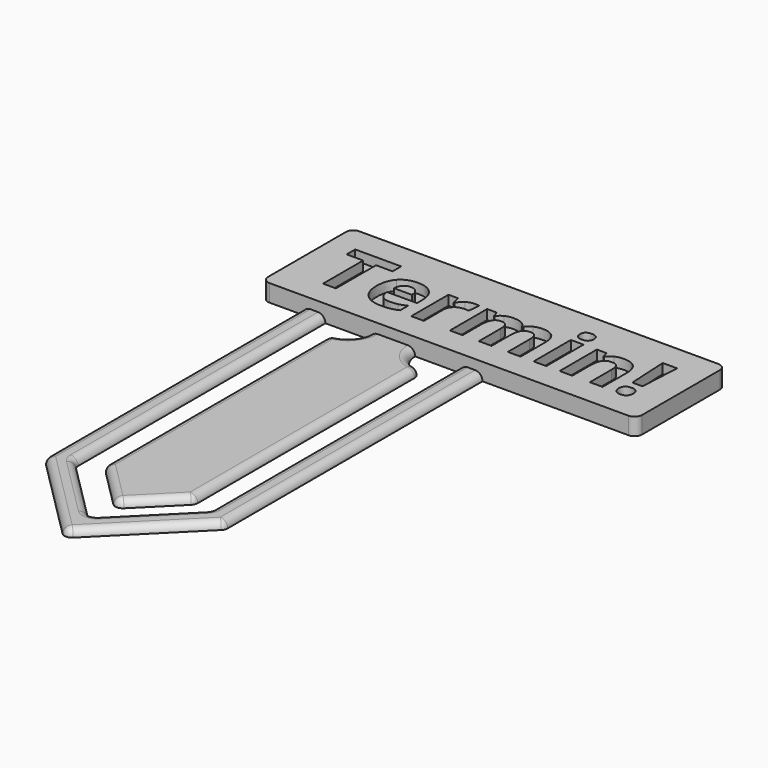
from build123d import *

# Parameters (mm, degrees)
F0_TEXT_SIZE = 11.3961958721
F1_DEPTH     = 1
F0_W         = 1.6969647916
F0_H         = 6.2216106839
F2_DEPTH     = 2.3
F3_R         = 0.99999


# Not quite as in the source:
# - a fillet or chamfer is up to 0.001 mm smaller than in the source, because OpenCascade refuses the exact size
# - Text() gives the source's letters only with a copy of the font that has no kerning and outlines rounded to 1/6400 em; it was checked with that copy


with BuildPart() as f1:
    # F0 (on Top) → F1 (new body)
    with BuildSketch(Plane.XY):
        Polygon((-11.1783012444, 18.0121831276), (-14.1783012444, 18.0121831276), (-14.1783012444, -24.9878168724), (-2.1783012444, -36.9878168724), (9.8216987556, -24.9878168724), (9.8216987556, 18.0121831276), (6.8216987556, 18.0121831276), (6.8216987556, -23.7451761852), (-2.1783012444, -32.7451761852), (-11.1783012444, -23.7451761852), align=None)
        with BuildLine():
            Line((0.8216987556, 18.0121831276), (-5.1783012444, 18.0121831276))
            ThreePointArc((-5.1783012444, 18.0121831276), (-6.0569809009, 15.8908627841), (-8.1783012444, 15.0121831276))
            Line((-8.1783012444, 15.0121831276), (-8.1783012444, -22.5025354981))
            Line((-8.1783012444, -22.5025354981), (-2.1783012444, -28.5025354981))
            Line((-2.1783012444, -28.5025354981), (3.8216987556, -22.5025354981))
            Line((3.8216987556, -22.5025354981), (3.8216987556, 15.0121831276))
            ThreePointArc((3.8216987556, 15.0121831276), (1.700378412, 15.8908627841), (0.8216987556, 18.0121831276))
        make_face()
        with Locations((-16.6529401391, 21.4095526137)):
            Text('Termin!', F0_TEXT_SIZE, font='Open Sans', font_style=FontStyle.BOLD, text_align=(TextAlign.LEFT, TextAlign.BOTTOM))
    extrude(amount=F1_DEPTH)

    # F0 (on Top) → F2 (join)
    with BuildSketch(Plane.XY):
        Polygon((-19.6529401391, 18.0121831276), (-14.1783012444, 18.0121831276), (-11.1783012444, 18.0121831276), (-5.1783012444, 18.0121831276), (0.8216987556, 18.0121831276), (6.8216987556, 18.0121831276), (9.8216987556, 18.0121831276), (30.3470598609, 18.0121831276), (30.3470598609, 33.0121831276), (-19.6529401391, 33.0121831276), align=None)
        Polygon((-12.4897673346, 28.1101596554), (-12.4897673346, 21.4095526137), (-14.2152226158, 21.4095526137), (-14.2152226158, 28.1101596554), (-16.4250162217, 28.1101596554), (-16.4250162217, 29.545368073), (-10.2817543843, 29.545368073), (-10.2817543843, 28.1101596554), align=None, mode=Mode.SUBTRACT)
        with BuildLine():
            add(Edge.make_bspline(
                [(-5.112511163, 21.4059913025), (-5.6182173548, 21.2973713106), (-6.3482861529, 21.2973713106)],
                knots=[0, 0, 0, 1, 1, 1], degree=2))
            add(Edge.make_bspline(
                [(-6.3482861529, 21.2973713106), (-7.8493788279, 21.2973713106), (-8.6951902403, 22.1271568225)],
                knots=[0, 0, 0, 1, 1, 1], degree=2))
            add(Edge.make_bspline(
                [(-8.6951902403, 22.1271568225), (-9.5410016527, 22.9569423344), (-9.5410016527, 24.4758415655)],
                knots=[0, 0, 0, 1, 1, 1], degree=2))
            add(Edge.make_bspline(
                [(-9.5410016527, 24.4758415655), (-9.5410016527, 26.0392571867), (-8.7592938421, 26.8930815493)],
                knots=[0, 0, 0, 1, 1, 1], degree=2))
            add(Edge.make_bspline(
                [(-8.7592938421, 26.8930815493), (-7.9775860314, 27.7469059119), (-6.5975779376, 27.7469059119)],
                knots=[0, 0, 0, 1, 1, 1], degree=2))
            add(Edge.make_bspline(
                [(-6.5975779376, 27.7469059119), (-5.2798927898, 27.7469059119), (-4.5453723528, 26.9963595744)],
                knots=[0, 0, 0, 1, 1, 1], degree=2))
            add(Edge.make_bspline(
                [(-4.5453723528, 26.9963595744), (-3.8108519157, 26.2458132369), (-3.8108519157, 24.9210054668)],
                knots=[0, 0, 0, 1, 1, 1], degree=2))
            Line((-3.8108519157, 24.9210054668), (-3.8108519157, 24.0965619217))
            Line((-3.8108519157, 24.0965619217), (-7.8226689938, 24.0965619217))
            add(Edge.make_bspline(
                [(-7.8226689938, 24.0965619217), (-7.7941785041, 23.373615746), (-7.393530993, 22.9676262681)],
                knots=[0, 0, 0, 1, 1, 1], degree=2))
            add(Edge.make_bspline(
                [(-7.393530993, 22.9676262681), (-6.9928834819, 22.5616367901), (-6.2699373062, 22.5616367901)],
                knots=[0, 0, 0, 1, 1, 1], degree=2))
            add(Edge.make_bspline(
                [(-6.2699373062, 22.5616367901), (-5.7072501351, 22.5616367901), (-5.20688591, 22.6782697323)],
                knots=[0, 0, 0, 1, 1, 1], degree=2))
            add(Edge.make_bspline(
                [(-5.20688591, 22.6782697323), (-4.706521685, 22.7949026744), (-4.1616410699, 23.0513170815)],
                knots=[0, 0, 0, 1, 1, 1], degree=2))
            Line((-4.1616410699, 23.0513170815), (-4.1616410699, 21.737193245))
            add(Edge.make_bspline(
                [(-4.1616410699, 21.737193245), (-4.6068049711, 21.5146112944), (-5.112511163, 21.4059913025)],
                knots=[0, 0, 0, 1, 1, 1], degree=2))
        make_face(mode=Mode.SUBTRACT)
        with BuildLine():
            add(Edge.make_bspline(
                [(-0.0296297384, 27.4272782308), (0.4627215363, 27.7469059119), (1.041434608, 27.7469059119)],
                knots=[0, 0, 0, 1, 1, 1], degree=2))
            add(Edge.make_bspline(
                [(1.041434608, 27.7469059119), (1.3868817953, 27.7469059119), (1.6148057128, 27.697047555)],
                knots=[0, 0, 0, 1, 1, 1], degree=2))
            Line((1.6148057128, 27.697047555), (1.4865985092, 26.1069220997))
            add(Edge.make_bspline(
                [(1.4865985092, 26.1069220997), (1.280042459, 26.1621224235), (0.9862342842, 26.1621224235)],
                knots=[0, 0, 0, 1, 1, 1], degree=2))
            add(Edge.make_bspline(
                [(0.9862342842, 26.1621224235), (0.1742553283, 26.1621224235), (-0.279811851, 25.7445586841)],
                knots=[0, 0, 0, 1, 1, 1], degree=2))
            add(Edge.make_bspline(
                [(-0.279811851, 25.7445586841), (-0.7338790302, 25.3269949447), (-0.7338790302, 24.5755582794)],
                knots=[0, 0, 0, 1, 1, 1], degree=2))
            Line((-0.7338790302, 24.5755582794), (-0.7338790302, 21.4095526137))
            Line((-0.7338790302, 21.4095526137), (-2.4308438218, 21.4095526137))
            Line((-2.4308438218, 21.4095526137), (-2.4308438218, 27.6311632976))
            Line((-2.4308438218, 27.6311632976), (-1.145210475, 27.6311632976))
            Line((-1.145210475, 27.6311632976), (-0.8941380347, 26.5841378019))
            Line((-0.8941380347, 26.5841378019), (-0.8122278769, 26.5841378019))
            add(Edge.make_bspline(
                [(-0.8122278769, 26.5841378019), (-0.5219810132, 27.1076505497), (-0.0296297384, 27.4272782308)],
                knots=[0, 0, 0, 1, 1, 1], degree=2))
        make_face(mode=Mode.SUBTRACT)
        with BuildLine():
            Line((8.3136320989, 24.5310418893), (8.3136320989, 21.4095526137))
            Line((8.3136320989, 21.4095526137), (6.6166673073, 21.4095526137))
            Line((6.6166673073, 21.4095526137), (6.6166673073, 25.0438707035))
            add(Edge.make_bspline(
                [(6.6166673073, 25.0438707035), (6.6166673073, 25.7169585222), (6.3914143732, 26.0535024316)],
                knots=[0, 0, 0, 1, 1, 1], degree=2))
            add(Edge.make_bspline(
                [(6.3914143732, 26.0535024316), (6.1661614392, 26.3900463409), (5.6818231146, 26.3900463409)],
                knots=[0, 0, 0, 1, 1, 1], degree=2))
            add(Edge.make_bspline(
                [(5.6818231146, 26.3900463409), (5.0301031632, 26.3900463409), (4.7354046606, 25.9110499832)],
                knots=[0, 0, 0, 1, 1, 1], degree=2))
            add(Edge.make_bspline(
                [(4.7354046606, 25.9110499832), (4.4407061579, 25.4320536254), (4.4407061579, 24.3369504283)],
                knots=[0, 0, 0, 1, 1, 1], degree=2))
            Line((4.4407061579, 24.3369504283), (4.4407061579, 21.4095526137))
            Line((4.4407061579, 21.4095526137), (2.7437413664, 21.4095526137))
            Line((2.7437413664, 21.4095526137), (2.7437413664, 27.6311632976))
            Line((2.7437413664, 27.6311632976), (4.0400586468, 27.6311632976))
            Line((4.0400586468, 27.6311632976), (4.2679825643, 26.8352102422))
            Line((4.2679825643, 26.8352102422), (4.3623573113, 26.8352102422))
            add(Edge.make_bspline(
                [(4.3623573113, 26.8352102422), (4.6134297516, 27.264348243), (5.0861938148, 27.5056270775)],
                knots=[0, 0, 0, 1, 1, 1], degree=2))
            add(Edge.make_bspline(
                [(5.0861938148, 27.5056270775), (5.5589578779, 27.7469059119), (6.171503406, 27.7469059119)],
                knots=[0, 0, 0, 1, 1, 1], degree=2))
            add(Edge.make_bspline(
                [(6.171503406, 27.7469059119), (7.5675374004, 27.7469059119), (8.0643403142, 26.8352102422)],
                knots=[0, 0, 0, 1, 1, 1], degree=2))
            Line((8.0643403142, 26.8352102422), (8.213915385, 26.8352102422))
            add(Edge.make_bspline(
                [(8.213915385, 26.8352102422), (8.4649878253, 27.2696902098), (8.9511068055, 27.5082980609)],
                knots=[0, 0, 0, 1, 1, 1], degree=2))
            add(Edge.make_bspline(
                [(8.9511068055, 27.5082980609), (9.4372257856, 27.7469059119), (10.0497713138, 27.7469059119)],
                knots=[0, 0, 0, 1, 1, 1], degree=2))
            add(Edge.make_bspline(
                [(10.0497713138, 27.7469059119), (11.1074807431, 27.7469059119), (11.6496903749, 27.2046962802)],
                knots=[0, 0, 0, 1, 1, 1], degree=2))
            add(Edge.make_bspline(
                [(11.6496903749, 27.2046962802), (12.1919000066, 26.6624866485), (12.1919000066, 25.4658860819)],
                knots=[0, 0, 0, 1, 1, 1], degree=2))
            Line((12.1919000066, 25.4658860819), (12.1919000066, 21.4095526137))
            Line((12.1919000066, 21.4095526137), (10.4895932482, 21.4095526137))
            Line((10.4895932482, 21.4095526137), (10.4895932482, 25.0438707035))
            add(Edge.make_bspline(
                [(10.4895932482, 25.0438707035), (10.4895932482, 25.7169585222), (10.2643403142, 26.0535024316)],
                knots=[0, 0, 0, 1, 1, 1], degree=2))
            add(Edge.make_bspline(
                [(10.2643403142, 26.0535024316), (10.0390873801, 26.3900463409), (9.5547490556, 26.3900463409)],
                knots=[0, 0, 0, 1, 1, 1], degree=2))
            add(Edge.make_bspline(
                [(9.5547490556, 26.3900463409), (8.9315195938, 26.3900463409), (8.6225758463, 25.9448824397)],
                knots=[0, 0, 0, 1, 1, 1], degree=2))
            add(Edge.make_bspline(
                [(8.6225758463, 25.9448824397), (8.3136320989, 25.4997185384), (8.3136320989, 24.5310418893)],
                knots=[0, 0, 0, 1, 1, 1], degree=2))
        make_face(mode=Mode.SUBTRACT)
        with Locations((14.7818635841, 24.5203579557)):
            Rectangle(F0_W, F0_H, mode=Mode.SUBTRACT)
        with BuildLine():
            add(Edge.make_bspline(
                [(14.7845345675, 28.4039678302), (13.8603743085, 28.4039678302), (13.8603743085, 29.239095309)],
                knots=[0, 0, 0, 1, 1, 1], degree=2))
            add(Edge.make_bspline(
                [(13.8603743085, 29.239095309), (13.8603743085, 30.0688808209), (14.7845345675, 30.0688808209)],
                knots=[0, 0, 0, 1, 1, 1], degree=2))
            add(Edge.make_bspline(
                [(14.7845345675, 30.0688808209), (15.7086948265, 30.0688808209), (15.7086948265, 29.239095309)],
                knots=[0, 0, 0, 1, 1, 1], degree=2))
            add(Edge.make_bspline(
                [(15.7086948265, 29.239095309), (15.7086948265, 28.8437897646), (15.4780999257, 28.6238787974)],
                knots=[0, 0, 0, 1, 1, 1], degree=2))
            add(Edge.make_bspline(
                [(15.4780999257, 28.6238787974), (15.2475050248, 28.4039678302), (14.7845345675, 28.4039678302)],
                knots=[0, 0, 0, 1, 1, 1], degree=2))
        make_face(mode=Mode.SUBTRACT)
        with BuildLine():
            add(Edge.make_bspline(
                [(24.9173552879, 21.507488672), (24.6618312085, 21.7549998011), (24.6618312085, 22.2055056691)],
                knots=[0, 0, 0, 1, 1, 1], degree=2))
            add(Edge.make_bspline(
                [(24.6618312085, 22.2055056691), (24.6618312085, 22.6720374376), (24.912013321, 22.9115356165)],
                knots=[0, 0, 0, 1, 1, 1], degree=2))
            add(Edge.make_bspline(
                [(24.912013321, 22.9115356165), (25.1621954335, 23.1510337954), (25.6411917913, 23.1510337954)],
                knots=[0, 0, 0, 1, 1, 1], degree=2))
            add(Edge.make_bspline(
                [(25.6411917913, 23.1510337954), (26.102381593, 23.1510337954), (26.3552346889, 22.9061936497)],
                knots=[0, 0, 0, 1, 1, 1], degree=2))
            add(Edge.make_bspline(
                [(26.3552346889, 22.9061936497), (26.6080877848, 22.661353504), (26.6080877848, 22.2055056691)],
                knots=[0, 0, 0, 1, 1, 1], degree=2))
            add(Edge.make_bspline(
                [(26.6080877848, 22.2055056691), (26.6080877848, 21.7656837347), (26.3525637055, 21.5128306388)],
                knots=[0, 0, 0, 1, 1, 1], degree=2))
            add(Edge.make_bspline(
                [(26.3525637055, 21.5128306388), (26.0970396262, 21.2599775429), (25.6411917913, 21.2599775429)],
                knots=[0, 0, 0, 1, 1, 1], degree=2))
            add(Edge.make_bspline(
                [(25.6411917913, 21.2599775429), (25.1728793672, 21.2599775429), (24.9173552879, 21.507488672)],
                knots=[0, 0, 0, 1, 1, 1], degree=2))
        make_face(mode=Mode.SUBTRACT)
        with BuildLine():
            Line((23.1536159111, 25.4658860819), (23.1536159111, 21.4095526137))
            Line((23.1536159111, 21.4095526137), (21.4566511195, 21.4095526137))
            Line((21.4566511195, 21.4095526137), (21.4566511195, 25.0438707035))
            add(Edge.make_bspline(
                [(21.4566511195, 25.0438707035), (21.4566511195, 25.7169585222), (21.2171529406, 26.0535024316)],
                knots=[0, 0, 0, 1, 1, 1], degree=2))
            add(Edge.make_bspline(
                [(21.2171529406, 26.0535024316), (20.9776547618, 26.3900463409), (20.4541420139, 26.3900463409)],
                knots=[0, 0, 0, 1, 1, 1], degree=2))
            add(Edge.make_bspline(
                [(20.4541420139, 26.3900463409), (19.7418797719, 26.3900463409), (19.4249230742, 25.9146112944)],
                knots=[0, 0, 0, 1, 1, 1], degree=2))
            add(Edge.make_bspline(
                [(19.4249230742, 25.9146112944), (19.1079663765, 25.4391762478), (19.1079663765, 24.3369504283)],
                knots=[0, 0, 0, 1, 1, 1], degree=2))
            Line((19.1079663765, 24.3369504283), (19.1079663765, 21.4095526137))
            Line((19.1079663765, 21.4095526137), (17.4110015849, 21.4095526137))
            Line((17.4110015849, 21.4095526137), (17.4110015849, 27.6311632976))
            Line((17.4110015849, 27.6311632976), (18.7073188654, 27.6311632976))
            Line((18.7073188654, 27.6311632976), (18.9352427828, 26.8352102422))
            Line((18.9352427828, 26.8352102422), (19.0296175299, 26.8352102422))
            add(Edge.make_bspline(
                [(19.0296175299, 26.8352102422), (19.3145224267, 27.2857161102), (19.8122156683, 27.5163110111)],
                knots=[0, 0, 0, 1, 1, 1], degree=2))
            add(Edge.make_bspline(
                [(19.8122156683, 27.5163110111), (20.3099089099, 27.7469059119), (20.9438223053, 27.7469059119)],
                knots=[0, 0, 0, 1, 1, 1], degree=2))
            add(Edge.make_bspline(
                [(20.9438223053, 27.7469059119), (22.0300222243, 27.7469059119), (22.5918190677, 27.1601798901)],
                knots=[0, 0, 0, 1, 1, 1], degree=2))
            add(Edge.make_bspline(
                [(22.5918190677, 27.1601798901), (23.1536159111, 26.5734538682), (23.1536159111, 25.4658860819)],
                knots=[0, 0, 0, 1, 1, 1], degree=2))
        make_face(mode=Mode.SUBTRACT)
        Polygon((26.6080877848, 29.545368073), (26.3249635436, 24.1090265109), (24.9681039726, 24.1090265109), (24.6831990758, 29.545368073), align=None, mode=Mode.SUBTRACT)
        with BuildLine():
            add(Edge.make_bspline(
                [(-5.7303986579, 26.1977355356), (-6.0473553556, 26.5396214117), (-6.5868940039, 26.5396214117)],
                knots=[0, 0, 0, 1, 1, 1], degree=2))
            add(Edge.make_bspline(
                [(-6.5868940039, 26.5396214117), (-7.1264326522, 26.5396214117), (-7.4327054163, 26.1977355356)],
                knots=[0, 0, 0, 1, 1, 1], degree=2))
            add(Edge.make_bspline(
                [(-7.4327054163, 26.1977355356), (-7.7389781804, 25.8558496594), (-7.7834945705, 25.2272782308)],
                knots=[0, 0, 0, 1, 1, 1], degree=2))
            Line((-7.7834945705, 25.2272782308), (-5.400977371, 25.2272782308))
            add(Edge.make_bspline(
                [(-5.400977371, 25.2272782308), (-5.4134419602, 25.8558496594), (-5.7303986579, 26.1977355356)],
                knots=[0, 0, 0, 1, 1, 1], degree=2))
        make_face()
    extrude(amount=F2_DEPTH)

    # F3 (radius 1 in the source; OpenCascade refuses exactly that, so slightly less here)
    f3_edges = [f1.edges().sort_by_distance(p)[0] for p in [
        (-19.65294, 18.012183, 1.15),
        (-19.65294, 33.012183, 1.15),
        (30.34706, 33.012183, 1.15),
        (30.34706, 18.012183, 1.15),
        (-2.178301, -36.987817, 0.5),
        (9.821699, -24.987817, 0.5),
        (-14.178301, -24.987817, 0.5),
        (-8.178301, -22.502535, 0.5),
        (-2.178301, -28.502535, 0.5),
        (3.821699, -22.502535, 0.5),
        (-8.178301, 15.012183, 0.5),
        (3.821699, 15.012183, 0.5),
        (3.821699, -30.987817, 1),
        (9.821699, -3.487817, 1),
        (-8.178301, -30.987817, 1),
        (-14.178301, -3.487817, 1),
        (3.821699, -3.745176, 1),
        (1.700378, 15.890863, 1),
        (-6.056981, 15.890863, 1),
        (-8.178301, -3.745176, 1),
        (-5.178301, -25.502535, 1),
        (0.821699, -25.502535, 1),
        (-11.178301, -23.745176, 0.5),
        (6.821699, -23.745176, 0.5),
        (-2.178301, -32.745176, 0.5),
        (2.321699, -28.245176, 1),
        (6.821699, -2.866497, 1),
        (-6.678301, -28.245176, 1),
        (-11.178301, -2.866497, 1),
    ]]
    fillet(f3_edges, radius=F3_R)


solid = f1.part
